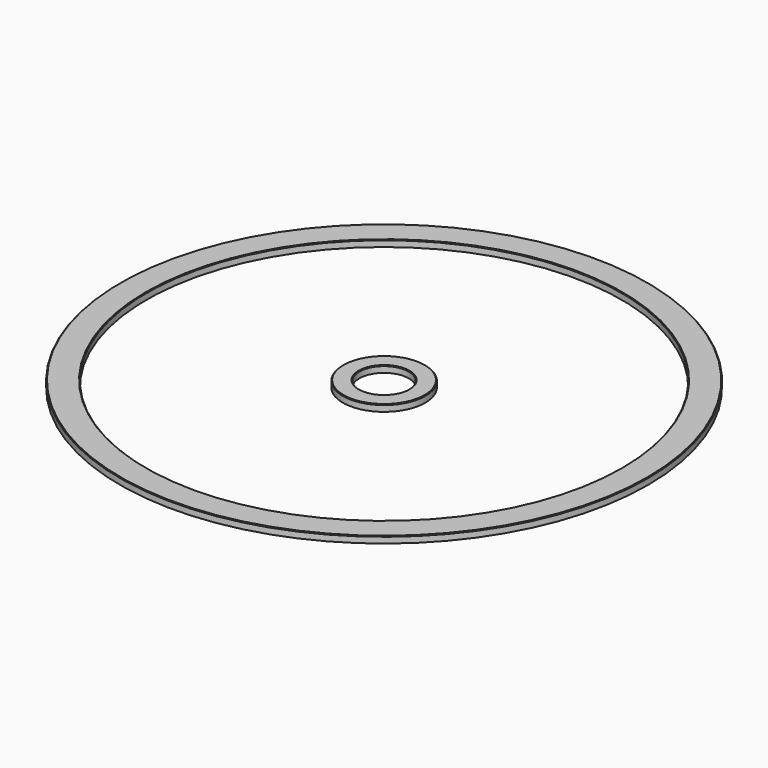
from build123d import *

# Parameters (mm, degrees)
F0_R     = 101.6
F1_DEPTH = 2.54
F2_R     = 9.525
F3_DEPTH = 25.4
F4_R     = 91.44
F4_R_2   = 15.875
F5_DEPTH = 2.541
F6_SIZE  = 0.254


with BuildPart() as f1:
    # F0 (on Top) → F1 (new body)
    with BuildSketch(Plane.XY):
        Circle(F0_R)
    extrude(amount=F1_DEPTH)

    # F2 (on face) → F3 (cut)
    with BuildSketch(Plane(origin=(0, 0, 0), x_dir=(1, 0, 0), z_dir=(0, 0, -1))):
        Circle(F2_R)
    extrude(amount=-F3_DEPTH, mode=Mode.SUBTRACT)

    # F4 (on face) → F5 (cut, through all)
    with BuildSketch(Plane.XY.offset(2.54)):
        Circle(F4_R)
        Circle(F4_R_2, mode=Mode.SUBTRACT)
    extrude(amount=-F5_DEPTH, mode=Mode.SUBTRACT)

    # F6
    f6_edges = [f1.edges().sort_by_distance(p)[0] for p in [
        (-101.6, 0, 2.54),
        (-91.44, 0, 2.54),
        (-15.875, 0, 2.54),
        (-9.525, 0, 2.54),
    ]]
    chamfer(f6_edges, length=F6_SIZE)


solid = f1.part
